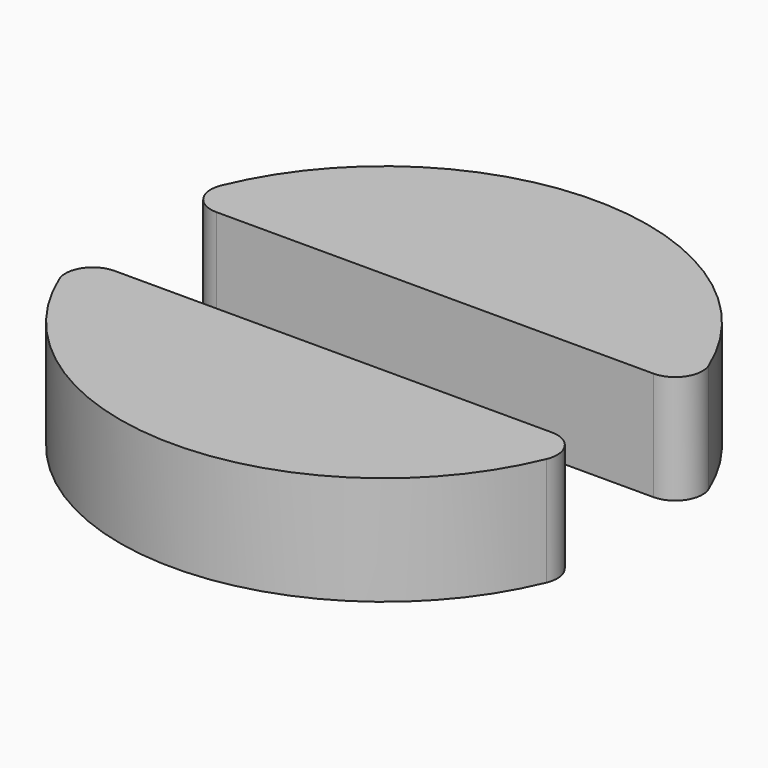
from build123d import *

# Parameters (mm, degrees)
F1_DEPTH = 20
F2_R     = 5
F2_2_R   = 5


with BuildPart() as f1:
    # F0 (on Top) → F1 (new body)
    with BuildSketch(Plane.XY):
        with BuildLine():
            Line((47.0879210033, -11.6936424747), (-47.0879210033, -11.6936424747))
            ThreePointArc((-47.0879210033, -11.6936424747), (0, -48.5181778176), (47.0879210033, -11.6936424747))
        make_face()
    extrude(amount=F1_DEPTH)

    # F2
    f2_edges = [f1.edges().sort_by_distance(p)[0] for p in [
        (-47.087921, -11.693642, 10),
        (47.087921, -11.693642, 10),
    ]]
    fillet(f2_edges, radius=F2_R)


with BuildPart() as f1b:
    # F0 (on Top) → F1, piece 2 (new body)
    with BuildSketch(Plane.XY):
        with BuildLine():
            ThreePointArc((47.0879210033, 11.6936424747), (0, 48.5181778176), (-47.0879210033, 11.6936424747))
            Line((-47.0879210033, 11.6936424747), (47.0879210033, 11.6936424747))
        make_face()
    extrude(amount=F1_DEPTH)

    # F2#2
    f2_2_edges = [f1b.edges().sort_by_distance(p)[0] for p in [
        (-47.087921, 11.693642, 10),
        (47.087921, 11.693642, 10),
    ]]
    fillet(f2_2_edges, radius=F2_2_R)


solid = Compound([f1.part, f1b.part])
